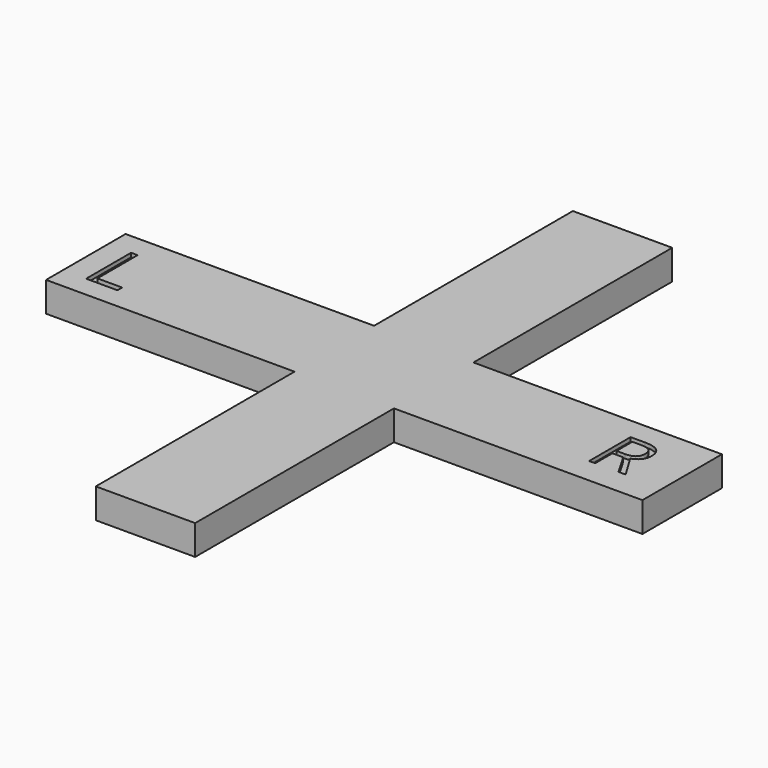
from build123d import *

# Parameters (mm, degrees)
F0_W           = 31.75
F0_H           = 12.7
F1_DEPTH       = 3.81
F2_TEXT_SIZE   = 10.0634018761
F2_TEXT_SIZE_2 = 9.2717741306
F3_DEPTH       = 0.508


# Not quite as in the source:
# - Text() gives the source's letters only with a copy of the font that has no kerning and outlines rounded to 1/6400 em; it was checked with that copy


with BuildPart() as f1:
    # F0 (on Top) → F1 (new body)
    with BuildSketch(Plane.XY):
        with Locations((-22.225, 0)):
            Rectangle(F0_W, F0_H)
        Polygon((-6.35, 6.35), (-6.35, -6.35), (0, -6.35), (6.35, -6.35), (6.35, 6.35), (0, 6.35), align=None)
        Polygon((0, -6.35), (-6.35, -6.35), (-6.35, -38.1), (6.35, -38.1), (6.35, -6.35), align=None)
        Polygon((-6.35, 38.1), (-6.35, 6.35), (0, 6.35), (6.35, 6.35), (6.35, 38.1), align=None)
        with Locations((22.225, 0)):
            Rectangle(F0_W, F0_H)
    extrude(amount=F1_DEPTH)

    # F2 (on face) → F3 (cut)
    with BuildSketch(Plane.XY.offset(3.81)):
        with Locations((-36.1270494759, -3.6557116546)):
            Text('L', F2_TEXT_SIZE, font='Open Sans', text_align=(TextAlign.LEFT, TextAlign.BOTTOM))
        with Locations((27.7574434876, -3.0691162683)):
            Text('R', F2_TEXT_SIZE_2, font='Open Sans', text_align=(TextAlign.LEFT, TextAlign.BOTTOM))
    extrude(amount=-F3_DEPTH, mode=Mode.SUBTRACT)


solid = f1.part
